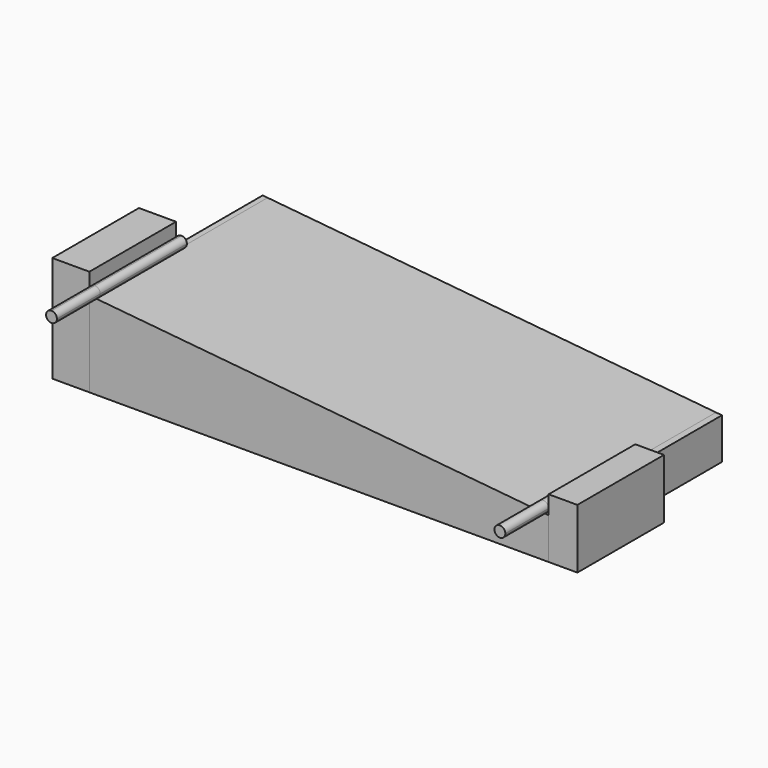
from build123d import *

# Parameters (mm, degrees)
F1_DEPTH      = 100
F2_DEPTH      = 25
F2_DEPTH_BACK = 50
F4_DEPTH      = 50


with BuildPart() as f1:
    # F0 (on Front) → F1 (new body)
    with BuildSketch(Plane.XZ):
        Polygon((0, 39.4), (0, 0), (212, 0), (212, 18.9867217821), (209.2603855849, 19.2505166466), (2.2603855436, 39.1823496275), align=None)
    extrude(amount=-F1_DEPTH)


with BuildPart() as f2:
    # F0 (on Front) → F2 (new body, two sides)
    with BuildSketch(Plane.XZ) as f2_sk:
        with BuildLine():
            ThreePointArc((2.5, 44.1708401161), (0.0028790356, 41.7907854751), (2.2603855436, 39.1823496275))
            ThreePointArc((2.2603855436, 39.1823496275), (4.1809169907, 39.820294772), (5, 41.6708401161))
            ThreePointArc((5, 41.6708401161), (4.267766953, 43.4386070691), (2.5, 44.1708401161))
        make_face()
    extrude(amount=F2_DEPTH)
    extrude(f2_sk.sketch, amount=-F2_DEPTH_BACK)


with BuildPart() as f2b:
    # F0 (on Front) → F2, piece 2 (new body, two sides)
    with BuildSketch(Plane.XZ) as f2_2_sk:
        with BuildLine():
            ThreePointArc((212, 21.7390071392), (207.819082994, 23.5895524694), (209.2603855849, 19.2505166466))
            ThreePointArc((209.2603855849, 19.2505166466), (211.180917006, 19.8884618091), (212, 21.7390071392))
        make_face()
    extrude(amount=F2_DEPTH)
    extrude(f2_2_sk.sketch, amount=-F2_DEPTH_BACK)


with BuildPart() as f4:
    # F3 (on face) → F4 (new body)
    with BuildSketch(Plane.XZ):
        Polygon((-17.1377528459, 0), (0, 0), (0, 39.4), (0, 49.0273796022), (-17.1377528459, 49.0273796022), align=None)
    extrude(amount=-F4_DEPTH)


with BuildPart() as f4b:
    # F3 (on face) → F4, piece 2 (new body)
    with BuildSketch(Plane.XZ):
        Polygon((212, 18.9867217821), (212, 0), (225.2641618252, 0), (225.2641618252, 27.517311275), (212, 27.517311275), align=None)
    extrude(amount=-F4_DEPTH)


solid = Compound([f1.part, f2.part, f2b.part, f4.part, f4b.part])
